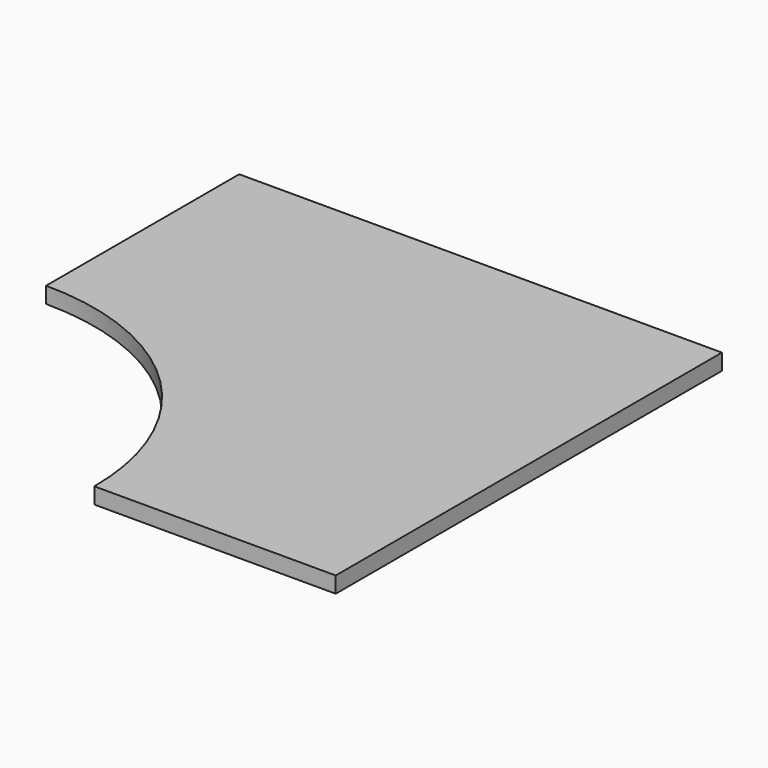
from build123d import *

# Parameters (mm, degrees)
F1_DEPTH = 40


# Not quite as in the source:
# - a feature names something its author has since deleted; it is built from what else it names


with BuildPart() as f1:
    # F0 (on Top) → F1 (new body)
    with BuildSketch(Plane.XY):
        with BuildLine():
            Line((0, -600), (600, -600))
            Line((600, -600), (600, 600))
            Line((600, 600), (-600, 600))
            Line((-600, 600), (-600, 0))
            ThreePointArc((-600, 0), (-175.7359312881, -175.7359312881), (0, -600))
        make_face()
    extrude(amount=F1_DEPTH)


solid = f1.part
